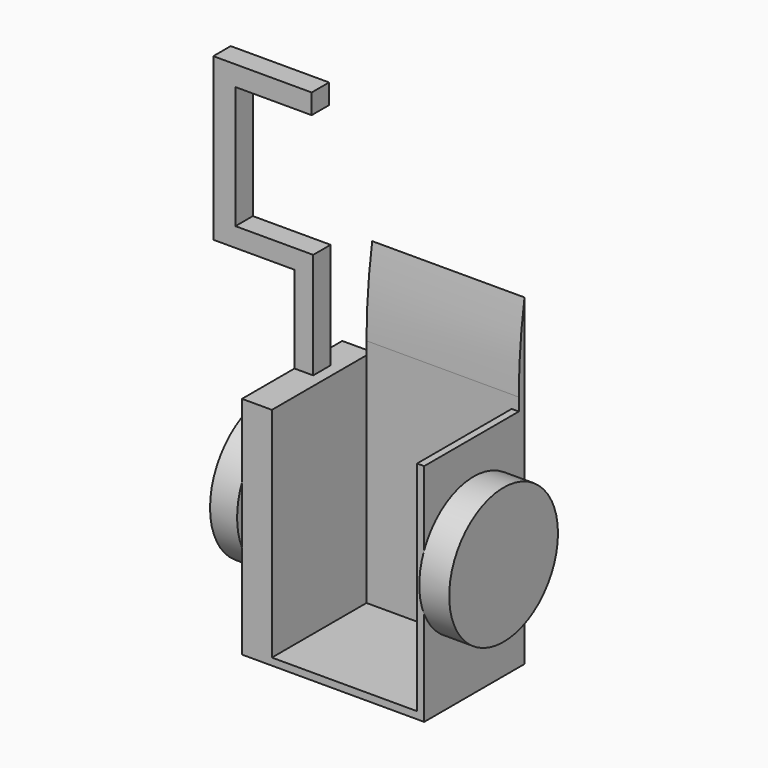
from build123d import *

# Parameters (mm, degrees)
F0_W         = 64.9794517085
F0_H         = 80.3038775921
F1_DEPTH     = 44.704
F2_T         = -2.54
F3_R         = 24.241575959
F1_FACE1_W   = 44.704
F1_FACE1_H   = 80.3038775921
F4_DEPTH     = 10.668
F5_R         = 25.1594880742
F6_DEPTH     = 9.652
F7_W         = 6.6666891798
F7_H         = 7.7688368037
F8_DEPTH     = 37.846
F9_W         = 7.7688368037
F9_H         = 6.8424391291
F10_DEPTH    = 28.956
F11_W        = 7.8935802502
F11_H        = 7.7688368037
F12_DEPTH    = 25.4
F13_DEPTH    = 25.4
F15_DEPTH    = 34.798
F16_T1_DEPTH = 205.6075505485
F17_W        = 7.7688368037
F17_H        = 7.1335003994
F18_DEPTH    = 27.178


# Not quite as in the source:
# - a fillet or chamfer that OpenCascade refuses, or shapes differently, is made with other operations: its cross-section is extruded or revolved along the edge and cut away or added


with BuildPart() as f1:
    # F0 (on Front) → F1 (new body)
    with BuildSketch(Plane.XZ):
        with Locations((25.8230366744, -3.7049613893)):
            Rectangle(F0_W, F0_H)
    extrude(amount=F1_DEPTH)

    # F2
    f2_openings = [f1.faces().sort_by_distance(p)[0] for p in [
        (25.823037, -22.352, 36.446977),
        (25.823037, -44.704, -3.704961),
    ]]
    offset(amount=F2_T, openings=f2_openings)

    # F3 (on face) + F1_face1 (on face) → F4 (join)
    with BuildSketch(Plane.YZ.offset(58.3127625287)):
        with Locations((-22.6588118821, 0)):
            Circle(F3_R)
    with BuildSketch(Plane(origin=(-6.6666891798, -22.352, -3.7049613893), x_dir=(0, -1, 0), z_dir=(-1, 0, 0))):
        Rectangle(F1_FACE1_W, F1_FACE1_H)
    extrude(amount=F4_DEPTH, dir=(1, 0, 0))

    # F5 (on face) → F6 (join)
    with BuildSketch(Plane(origin=(-6.6666891798, 0, 0), x_dir=(0, -1, 0), z_dir=(-1, 0, 0))):
        with Locations((21.7208880931, 0)):
            Circle(F5_R)
    extrude(amount=F6_DEPTH)

    # F7 (on face) → F8 (join)
    with BuildSketch(Plane.XY.offset(36.4469774067)):
        with Locations((-3.3333445899, -17.414805945)):
            Rectangle(F7_W, F7_H)
    extrude(amount=F8_DEPTH)

    # F9 (on face) → F10 (join)
    with BuildSketch(Plane(origin=(-6.6666891798, 0, 0), x_dir=(0, -1, 0), z_dir=(-1, 0, 0))):
        with Locations((17.414805945, 70.8717578422)):
            Rectangle(F9_W, F9_H)
    extrude(amount=F10_DEPTH)

    # F11 (on face) → F12 (join)
    with BuildSketch(Plane.XY.offset(74.2929774067)):
        with Locations((-31.6758990547, -17.414805945)):
            Rectangle(F11_W, F11_H)
    extrude(amount=F12_DEPTH)

    # F13 (add): a face of the model
    f13_faces = [f1.faces().sort_by_distance(p)[0] for p in [
        (-31.6758990547, -17.414805945, 99.6929774067),
    ]]
    extrude(f13_faces, amount=F13_DEPTH)

    # F14 (on face) → F15 (join)
    with BuildSketch(Plane.XY.offset(36.4469774067)):
        Polygon((58.3127625287, -2.54), (58.3127625287, 0), (4.0013108202, 0), (4.0013108202, -2.54), (55.7727625287, -2.54), align=None)
    extrude(amount=F15_DEPTH)

    # F16: fillet of radius 181.5102324735 on 1 edges, made by hand

    # F16_s2 → F16_t1 (cut)
    with BuildSketch(Plane.YZ.offset(-71.6467385999)):
        with BuildLine():
            ThreePointArc((0, 71.2449774067), (-1.903885347, 56.1685767196), (-2.54, 40.9857576387))
            Line((-2.54, 40.9857576387), (-2.54, 71.2449774067))
            Line((-2.54, 71.2449774067), (0, 71.2449774067))
        make_face()
    extrude(amount=F16_T1_DEPTH, mode=Mode.SUBTRACT)

    # F17 (on face) → F18 (join)
    with BuildSketch(Plane.YZ.offset(-27.7291089296)):
        with Locations((-17.414805945, 121.5262272071)):
            Rectangle(F17_W, F17_H)
    extrude(amount=F18_DEPTH)


solid = f1.part
